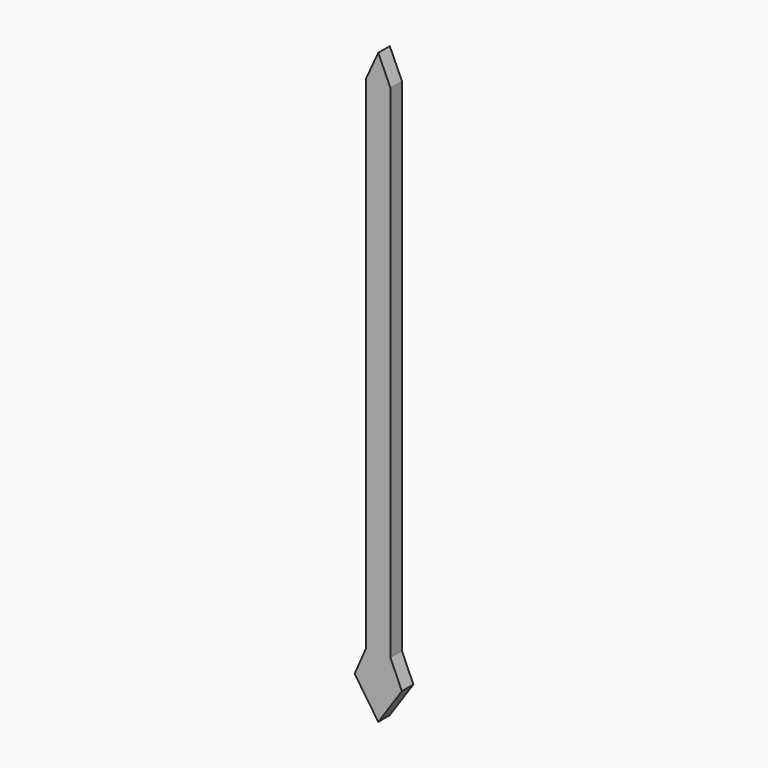
from build123d import *
from build123d import SkipClean  # not in build123d's __all__

# Parameters (mm, degrees)
F1_DEPTH = 6.35
F2_DEPTH = 6.35
F3_SIZE2 = 6.34999
F3_SIZE  = 6.34999
F4_DEPTH = 0.0254
F5_DEPTH = 0.0254
F7_DEPTH = 25.4
F8_DEPTH = 0.0254
F9_DEPTH = 0.0254


# Not quite as in the source:
# - a fillet or chamfer is up to 0.001 mm smaller than in the source, because OpenCascade refuses the exact size
# - ends of sketch curves that miss each other by under 0.0002 mm in the source are joined


with BuildPart() as f1:
    # F0 (on Front) → F1 (new body)
    with BuildSketch(Plane.XZ):
        Polygon((-17.139416188, 28.1973872334), (-27.9807504267, 3.4191238228), (0, -37.7674587071), (27.964355424, 3.4191238228), (17.08493568, 28.1973872334), (17.08493568, 469.1244959831), (0, 506.7884922028), (-17.139416188, 469.1244959831), align=None)
    extrude(amount=F1_DEPTH)

    # F2 (add): a face of the model
    f2_faces = [f1.faces().sort_by_distance(p)[0] for p in [
        (-0.0248835797, 0, 225.9211420486),
    ]]
    extrude(f2_faces, amount=F2_DEPTH)

    # F3 (size 6.35 and 6.35 in the source; OpenCascade refuses exactly that, so slightly less here)
    f3_edges = [f1.edges().sort_by_distance(p)[0] for p in [
        (-22.560083, -6.35, 15.808256),
        (-13.990375, -6.35, -17.174167),
        (13.982178, -6.35, -17.174167),
        (22.524646, -6.35, 15.808256),
        (17.084936, -6.35, 248.660942),
        (8.542468, -6.35, 487.956494),
        (-8.569708, -6.35, 487.956494),
        (-17.139416, -6.35, 248.660942),
        (-22.560083, 6.35, 15.808256),
        (-13.990375, 6.35, -17.174167),
        (13.982178, 6.35, -17.174167),
        (22.524646, 6.35, 15.808256),
        (17.084936, 6.35, 248.660942),
        (8.542468, 6.35, 487.956494),
        (-8.569708, 6.35, 487.956494),
        (-17.139416, 6.35, 248.660942),
    ]]
    chamfer(f3_edges, length=F3_SIZE, length2=F3_SIZE2)

    # F4 (add): a face of the model
    f4_faces = [f1.faces().sort_by_distance(p)[0] for p in [
        (-0.0252861091, -6.35, 223.0026633937),
    ]]
    extrude(f4_faces, amount=F4_DEPTH)

    # F5 (add): a face of the model
    f5_faces = [f1.faces().sort_by_distance(p)[0] for p in [
        (-0.0252861091, 6.35, 223.0026633937),
    ]]
    extrude(f5_faces, amount=F5_DEPTH)

    # F6 (on face) → F7 (cut)
    with BuildSketch(Plane.XZ.offset(6.3754)):
        Polygon((10.73493568, 467.7515936734), (10.73493568, 99.0661755204), (32.7086560428, 99.0661755204), (32.7086560428, 505.495429039), (10.73493568, 505.495429039), (10.73493568, 501.6054906496), (19.4450523704, 491.0283088684), (13.1097852611, 474.0980863571), (20.738528953, 474.0980863571), (20.738528953, 467.7515928086), align=None)
        Polygon((32.7086560428, 99.0661755204), (10.73493568, 99.0661755204), (10.73493568, 29.554810375), (20.738528953, 31.6301956773), (21.6034320424, 29.554810375), (32.7086560428, 29.554810375), align=None)
        Polygon((20.738528953, 31.6301956773), (10.73493568, 29.554810375), (21.6034320424, 29.554810375), align=None)
        Polygon((21.6034320424, 29.554810375), (10.73493568, 29.554810375), (10.73493568, 26.8647358603), (20.738530435, 4.0811948515), (27.3526439581, -1.5923568075), (32.2193913162, 4.0811982268), align=None)
        Polygon((-0.0092029974, 491.4372314137), (10.73494568, 467.7515949707), (10.73493568, 474.0980863571), (10.73493568, 501.6054906496), (0, 514.6415233612), (-11.796230803, 486.6769015789), (-10.789416188, 486.6769015789), (-10.789416188, 467.7476089999), align=None)
        Polygon((13.1097852611, 474.0980863571), (10.73493568, 467.7515928086), (20.738528953, 467.7515928086), (20.738528953, 474.0980863571), align=None)
        Polygon((10.73493568, 474.0980863571), (10.73493568, 467.7515936734), (13.1097852611, 474.0980863571), align=None)
        Polygon((10.73493568, 501.6054906496), (10.73493568, 474.0980863571), (13.1097852611, 474.0980863571), (19.4450523704, 491.0283088684), align=None)
        Polygon((27.3526439581, -1.5923568075), (20.738528953, 4.0811982268), (24.6255261009, -4.7715753101), align=None)
        Polygon((24.6255261009, -4.7715753101), (20.738530435, 4.0811948515), (-0.0015394217, -26.4652965043), (0, -41.624262929), (29.7397422671, -3.639997893), (27.3526439581, -1.5923568075), align=None)
        Polygon((-16.2565966219, 476.1029779911), (-10.789416188, 467.7476075543), (-10.789416188, 486.6769015789), (-11.796230803, 486.6769015789), align=None)
        Polygon((-10.789416188, 26.8690092904), (-10.789416188, 467.7476089999), (-16.2565966219, 476.1029779911), (-11.796230803, 486.6769015789), (-21.7237770557, 486.6769015789), (-21.7237770557, 26.8690092904), (-20.8278130876, 26.8690092904), (-18.3457657695, 33.1129990518), align=None)
        Polygon((0, -41.624262929), (-0.0015394241, -26.4652787056), (-20.7574730934, 4.0866529625), (-30.316057774, 2.9998017031), align=None)
        Polygon((-20.8278130876, 26.8690092904), (-10.789416188, 26.8690092904), (-18.3457657695, 33.1129990518), align=None)
        Polygon((-20.7574730934, 4.0866529625), (-10.789416188, 26.8690092904), (-20.8278130876, 26.8690092904), (-30.316057774, 2.9998017031), align=None)
    with SkipClean():  # cleaning this boolean's faces spoils the solid; the shape is the same uncleaned
        extrude(amount=-F7_DEPTH, mode=Mode.SUBTRACT)

    # F8 (cut): a face of the model
    f8_faces = [f1.faces().sort_by_distance(p)[0] for p in [
        (-0.0252861091, -6.3754, 223.0026633937),
    ]]
    extrude(f8_faces, amount=-F8_DEPTH, mode=Mode.SUBTRACT)

    # F9 (cut): a face of the model
    f9_faces = [f1.faces().sort_by_distance(p)[0] for p in [
        (-0.0252864299, 6.3754, 223.0026587516),
    ]]
    extrude(f9_faces, amount=-F9_DEPTH, mode=Mode.SUBTRACT)


solid = f1.part
